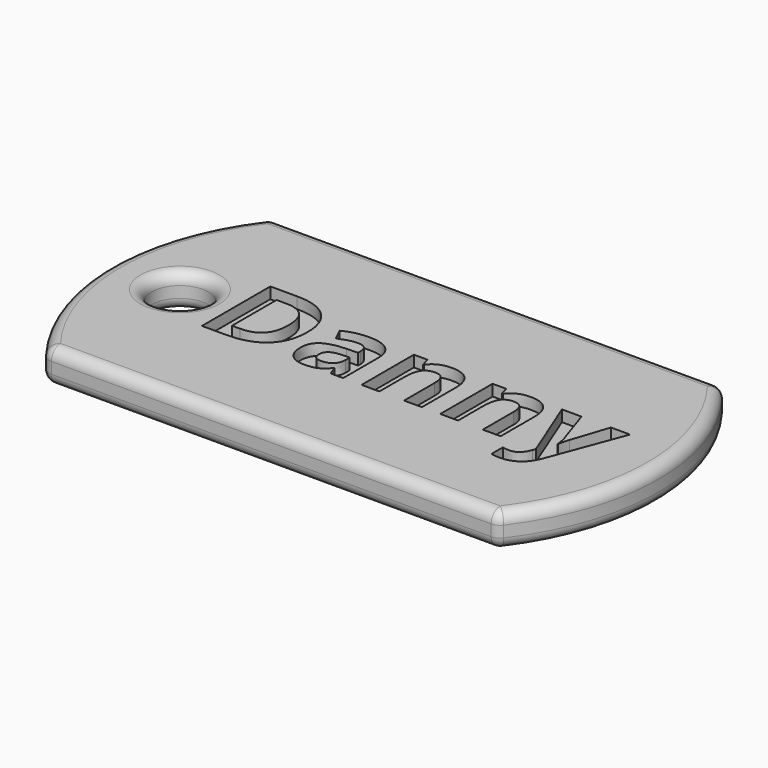
from build123d import *

# Parameters (mm, degrees)
F0_R         = 2.5
F1_DEPTH     = 3
F2_TEXT_SIZE = 10.6302201974
F3_DEPTH     = 1
F4_TEXT_SIZE = 11.5356885364
F5_DEPTH     = 1
F6_R         = 1


# Not quite as in the source:
# - Text() gives the source's letters only with a copy of the font that has no kerning and outlines rounded to 1/6400 em; it was checked with that copy


with BuildPart() as f1:
    # F0 (on Top) → F1 (new body)
    with BuildSketch(Plane.XY):
        with BuildLine():
            Line((20, 12.5), (-20, 12.5))
            ThreePointArc((-20, 12.5), (-24.387505004, 0), (-20, -12.5))
            Line((-20, -12.5), (20, -12.5))
            ThreePointArc((20, -12.5), (24.387505004, 0), (20, 12.5))
        make_face()
        with Locations((-18.112494996, 0)):
            Circle(F0_R, mode=Mode.SUBTRACT)
    extrude(amount=F1_DEPTH)

    # F2 (on face) → F3 (cut)
    with BuildSketch(Plane.XY.offset(3)):
        with Locations((-14.4549424787, -3.3249218556)):
            Text('Danny', F2_TEXT_SIZE, font='Open Sans', font_style=FontStyle.BOLD, text_align=(TextAlign.LEFT, TextAlign.BOTTOM))
    extrude(amount=-F3_DEPTH, mode=Mode.SUBTRACT)

    # F4 (on face) → F5 (cut)
    with BuildSketch(Plane(origin=(0, 0, 0), x_dir=(1, 0, 0), z_dir=(0, 0, -1))):
        with Locations((-13.4398699892, -3.8352218119)):
            Text('Braun', F4_TEXT_SIZE, font='Open Sans', font_style=FontStyle.BOLD, text_align=(TextAlign.LEFT, TextAlign.BOTTOM))
    extrude(amount=-F5_DEPTH, mode=Mode.SUBTRACT)

    # F6
    f6_edges = [f1.edges().sort_by_distance(p)[0] for p in [
        (20, -12.5, 1.5),
        (20, 12.5, 1.5),
        (24.387505, 0, 0),
        (24.387505, 0, 3),
        (-20, -12.5, 1.5),
        (0, -12.5, 0),
        (0, -12.5, 3),
        (-15.612495, 0, 1.5),
        (-20.612495, 0, 0),
        (-20.612495, 0, 3),
        (-20, 12.5, 1.5),
        (-24.387505, 0, 0),
        (-24.387505, 0, 3),
        (0, 12.5, 0),
        (0, 12.5, 3),
    ]]
    fillet(f6_edges, radius=F6_R)


solid = f1.part
